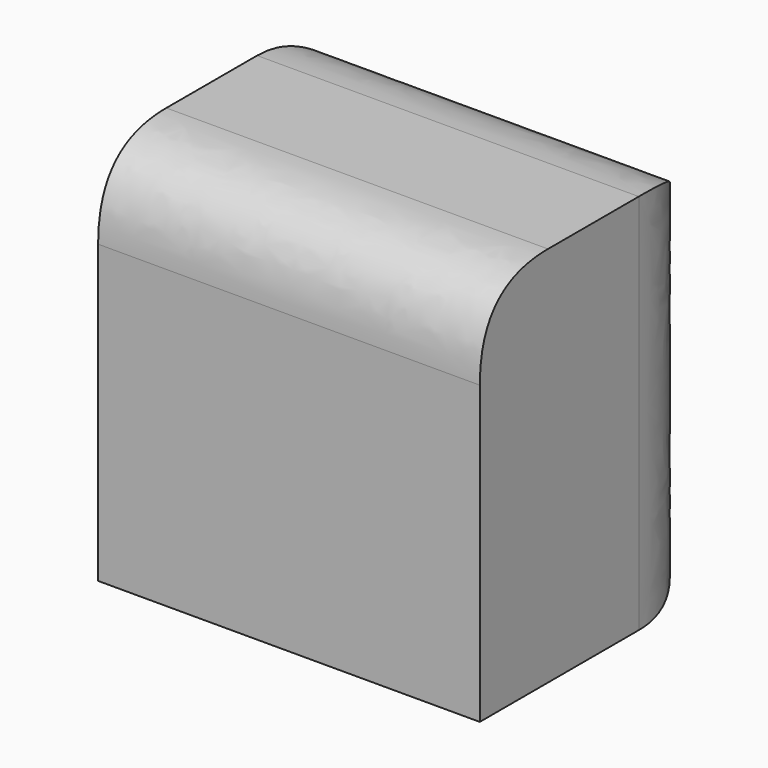
from build123d import *

# Parameters (mm, degrees)
F0_W        = 101.6
F0_H        = 101.6
F1_DEPTH    = 76.2
F2_T1_DEPTH = 215.0438952959
F3_T1_DEPTH = 218.1099465201
F3_T3_DEPTH = 218.1099465201


# Not quite as in the source:
# - a fillet or chamfer that OpenCascade refuses, or shapes differently, is made with other operations: its cross-section is extruded or revolved along the edge and cut away or added


with BuildPart() as f1:
    # F0 (on Front) → F1 (new body)
    with BuildSketch(Plane.XZ):
        with Locations((0.8658623874, 6.5226784527)):
            Rectangle(F0_W, F0_H)
    extrude(amount=F1_DEPTH)

    # F2: fillet of radius 22.6887790592 on 1 edges, made by hand

    # F2_s2 → F2_t1 (cut)
    with BuildSketch(Plane.YZ.offset(-106.6560852605)):
        with BuildLine():
            add(Edge.make_bspline(
                [(-53.5112209408, 57.3226784527), (-76.2, 57.3226784527), (-76.2, 34.6338993935)],
                knots=[0, 0, 0, 1, 1, 1], degree=2, weights=[1, 1, 1]))
            Line((-76.2, 34.6338993935), (-76.2, 57.3226784527))
            Line((-76.2, 57.3226784527), (-53.5112209408, 57.3226784527))
        make_face()
    extrude(amount=F2_T1_DEPTH, mode=Mode.SUBTRACT)

    # F3: fillet of radius 23.301989304 on 4 edges, made by hand

    # F3_s2 → F3_t1 (cut)
    with BuildSketch(Plane.XY.offset(-102.5322948073)):
        with BuildLine():
            add(Edge.make_bspline(
                [(-49.9341376126, -23.301989304), (-49.9341376126, 0), (-26.6321483086, 0)],
                knots=[0, 0, 0, 1, 1, 1], degree=2, weights=[1, 1, 1]))
            Line((-26.6321483086, 0), (-49.9341376126, 0))
            Line((-49.9341376126, 0), (-49.9341376126, -23.301989304))
        make_face()
        with BuildLine():
            add(Edge.make_bspline(
                [(28.3638730834, 0), (51.6658623874, 0), (51.6658623874, -23.301989304)],
                knots=[0, 0, 0, 1, 1, 1], degree=2, weights=[1, 1, 1]))
            Line((51.6658623874, -23.301989304), (51.6658623874, 0))
            Line((51.6658623874, 0), (28.3638730834, 0))
        make_face()
    extrude(amount=F3_T1_DEPTH, mode=Mode.SUBTRACT)

    # F3_s4 → F3_t3 (cut)
    with BuildSketch(Plane.YZ.offset(-108.1891108726)):
        with BuildLine():
            add(Edge.make_bspline(
                [(0, -20.9753322432), (0, -44.2773215473), (-23.301989304, -44.2773215473)],
                knots=[0, 0, 0, 1, 1, 1], degree=2, weights=[1, 1, 1]))
            Line((-23.301989304, -44.2773215473), (0, -44.2773215473))
            Line((0, -44.2773215473), (0, -20.9753322432))
        make_face()
        with BuildLine():
            add(Edge.make_bspline(
                [(0, 34.0206891487), (0, 57.3226784527), (-23.301989304, 57.3226784527)],
                knots=[0, 0, 0, 1, 1, 1], degree=2, weights=[1, 1, 1]))
            Line((-23.301989304, 57.3226784527), (0, 57.3226784527))
            Line((0, 57.3226784527), (0, 34.0206891487))
        make_face()
    extrude(amount=F3_T3_DEPTH, mode=Mode.SUBTRACT)


solid = f1.part
